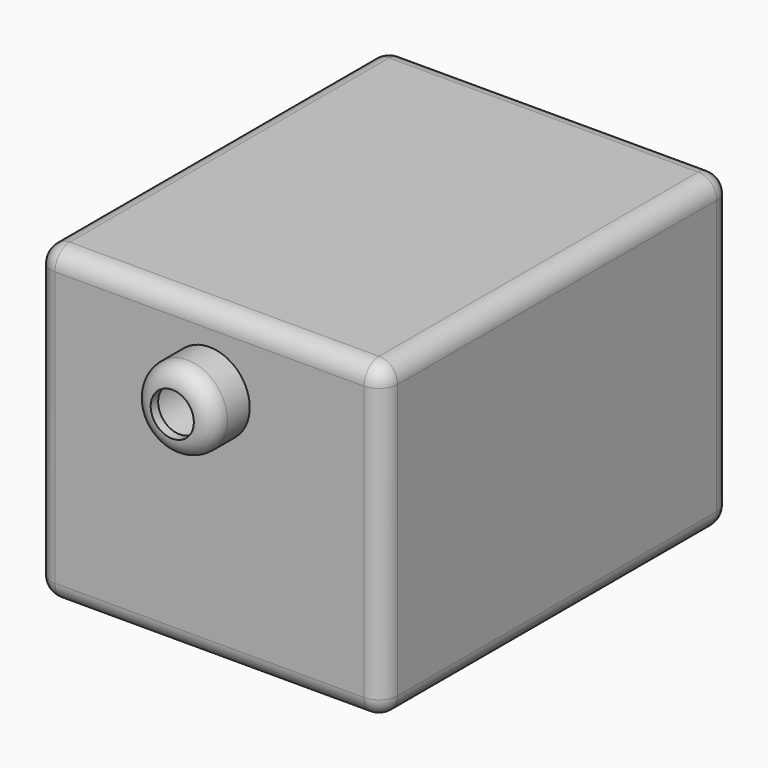
from build123d import *

# Parameters (mm, degrees)
F0_W     = 94.4138541818
F0_H     = 118.8927069306
F1_DEPTH = 84.88416
F2_R     = 10.9607963201
F3_DEPTH = 12.7
F4_R     = 5.08
F5_T     = -2.54


# Not quite as in the source:
# - a shell that OpenCascade refuses in one call is made with other operations: the cavity is built on its own and cut out


with BuildPart() as f1:
    # F0 (on Top) → F1 (new body)
    with BuildSketch(Plane.XY):
        Rectangle(F0_W, F0_H)
    extrude(amount=F1_DEPTH)

    # F2 (on face) → F3 (join)
    with BuildSketch(Plane.XZ.offset(59.4463534653)):
        with Locations((0, 64.512334764)):
            Circle(F2_R)
    extrude(amount=F3_DEPTH)

    # F4
    f4_edges = [f1.edges().sort_by_distance(p)[0] for p in [
        (0, -59.446353, 84.88416),
        (47.206927, 0, 84.88416),
        (47.206927, 0, 0),
        (0, -59.446353, 0),
        (0, 59.446353, 84.88416),
        (-47.206927, 0, 84.88416),
        (0, 59.446353, 0),
        (47.206927, 59.446353, 42.44208),
        (47.206927, -59.446353, 42.44208),
        (-47.206927, 59.446353, 42.44208),
        (-47.206927, 0, 0),
        (-47.206927, -59.446353, 42.44208),
        (-10.960796, -72.146353, 64.512335),
    ]]
    fillet(f4_edges, radius=F4_R)

    # F5: a shell. OpenCascade refuses it in one call, so the cavity is built on its own and cut out:
    # the body offset inwards by the wall thickness, plus a prism from it out through each open face.
    f5_core = offset(f1.part, amount=F5_T, kind=Kind.INTERSECTION, mode=Mode.PRIVATE)
    f5_exits = [f5_core.faces().sort_by_distance(p)[0] for p in [
        (0, -69.606353, 64.512335),
    ]]
    add(f5_core, mode=Mode.SUBTRACT)
    extrude(f5_exits, amount=-F5_T, mode=Mode.SUBTRACT)


solid = f1.part
